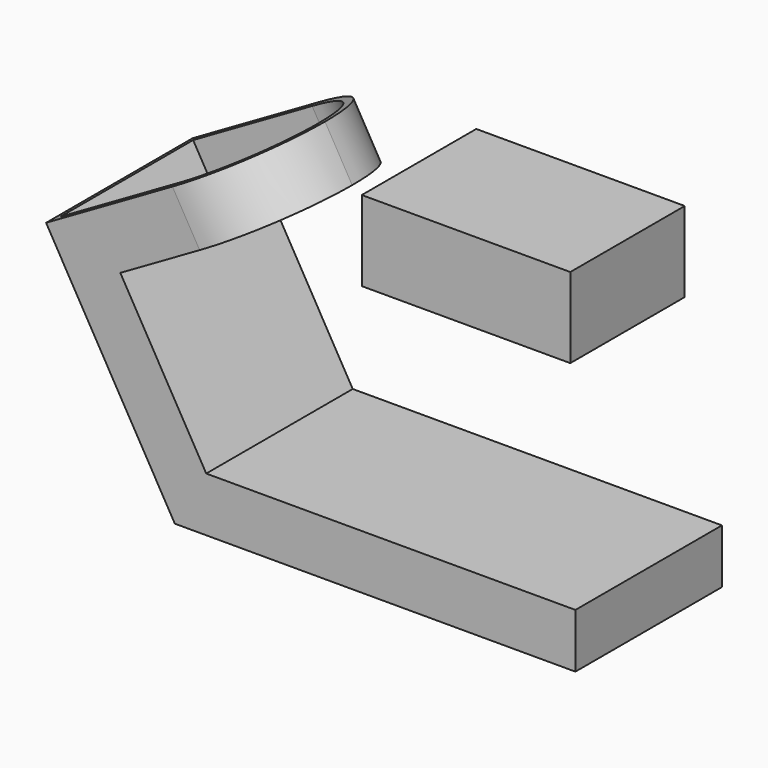
from build123d import *

# Parameters (mm, degrees)
F1_DEPTH = 32
F3_DEPTH = 19
F4_T     = -3
F5_R     = 9.5
F6_DEPTH = 3
F7_W     = 72.8673189878
F7_H     = 28.0379503965
F8_DEPTH = 50


# Not quite as in the source:
# - a feature names something its author has since deleted; it is built from what else it names


with BuildPart() as f1:
    # F0 (on Front) → F1 (new body, symmetric)
    with BuildSketch(Plane.XZ):
        Polygon((-45, 77.9422863406), (0, 0), (140, 0), (140, 19), (10.9696551146, 19), (-19.0455173281, 70.9878036687), (36.3801085141, 102.9878036687), (26.8801085141, 119.4422863406), align=None)
    extrude(amount=F1_DEPTH, both=True)

    # F2 (on face) → F3 (cut, through all)
    with BuildSketch(Plane(origin=(-45, 0, 77.9422863406), x_dir=(0.8660254038, 0, 0.5), z_dir=(-0.5, 0, 0.8660254038))):
        with BuildLine():
            Line((83, -32), (83, 0))
            ThreePointArc((83, 0), (73.627416998, -22.627416998), (51, -32))
            Line((51, -32), (83, -32))
        make_face()
        with BuildLine():
            ThreePointArc((51, 32), (73.627416998, 22.627416998), (83, 0))
            Line((83, 0), (83, 32))
            Line((83, 32), (51, 32))
        make_face()
    extrude(amount=-F3_DEPTH, mode=Mode.SUBTRACT)

    # F4
    f4_openings = [f1.faces().sort_by_distance(p)[0] for p in [
        (-11.74342, 0, 97.142982),
    ]]
    offset(amount=F4_T, openings=f4_openings, kind=Kind.INTERSECTION)

    # F5 (on face) → F6 (cut, through all)
    with BuildSketch(Plane(origin=(-37, 0, 64.08587988), x_dir=(0.8660254038, 0, 0.5), z_dir=(-0.5, 0, 0.8660254038))):
        with Locations((51, 0)):
            Circle(F5_R)
    extrude(amount=-F6_DEPTH, mode=Mode.SUBTRACT)


with BuildPart() as f8:
    # F7 (on Front) → F8 (new body)
    with BuildSketch(Plane.XZ):
        with Locations((116.1752715707, 120.3569099307)):
            Rectangle(F7_W, F7_H)
    extrude(amount=F8_DEPTH)


solid = Compound([f1.part, f8.part])
